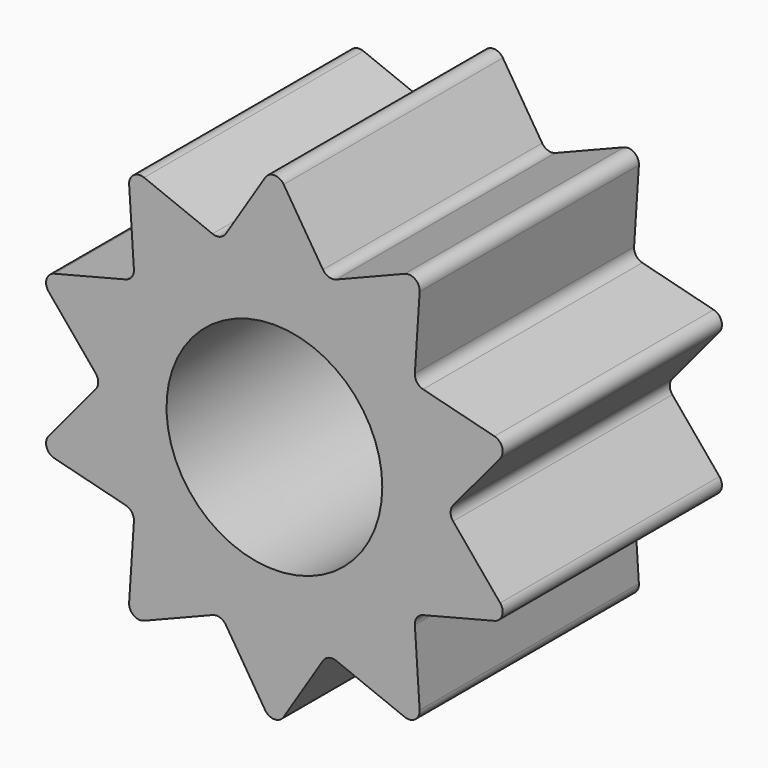
from build123d import *

# Parameters (mm, degrees)
F1_DEPTH = 2.54
F2_R     = 0.1016


# Not quite as in the source:
# - a feature names something its author has since deleted; it is built from what else it names


with BuildPart() as f1:
    # F0 (on Front) → F1 (new body)
    with BuildSketch(Plane.XZ):
        Polygon((0, 2.3086211489), (-0.4952492845, 1.5242205696), (-1.3569734644, 1.867713743), (-1.2965794597, 0.9420201184), (-2.1956291873, 0.7134031686), (-1.6026603504, 0), (-2.1956291873, -0.7134031686), (-1.2965794597, -0.9420201184), (-1.3569734644, -1.867713743), (-0.4952492845, -1.5242205696), (0, -2.3086211489), (0.4952492845, -1.5242205696), (1.3569734644, -1.867713743), (1.2965794597, -0.9420201184), (2.1956291873, -0.7134031686), (1.6026603504, 0), (2.1956291873, 0.7134031686), (1.2965794597, 0.9420201184), (1.3569734644, 1.867713743), (0.4952492845, 1.5242205696), align=None)
        with BuildLine():
            ThreePointArc((0, 1.00000054), (0.707107163, 0.707107163), (1.00000054, 0))
            ThreePointArc((1.00000054, 0), (-0.707107163, -0.707107163), (0, 1.00000054))
        make_face(mode=Mode.SUBTRACT)
    extrude(amount=F1_DEPTH)

    # F2
    f2_edges = [f1.edges().sort_by_distance(p)[0] for p in [
        (0, -1.27, 2.308621),
        (0.495249, -1.27, 1.524221),
        (1.356973, -1.27, 1.867714),
        (1.296579, -1.27, 0.94202),
        (2.195629, -1.27, 0.713403),
        (1.60266, -1.27, 0),
        (2.195629, -1.27, -0.713403),
        (1.296579, -1.27, -0.94202),
        (1.356973, -1.27, -1.867714),
        (0.495249, -1.27, -1.524221),
        (0, -1.27, -2.308621),
        (-1.356973, -1.27, -1.867714),
        (-0.495249, -1.27, -1.524221),
        (-1.296579, -1.27, -0.94202),
        (-2.195629, -1.27, -0.713403),
        (-1.60266, -1.27, 0),
        (-2.195629, -1.27, 0.713403),
        (-1.296579, -1.27, 0.94202),
        (-1.356973, -1.27, 1.867714),
        (-0.495249, -1.27, 1.524221),
    ]]
    fillet(f2_edges, radius=F2_R)


solid = f1.part
